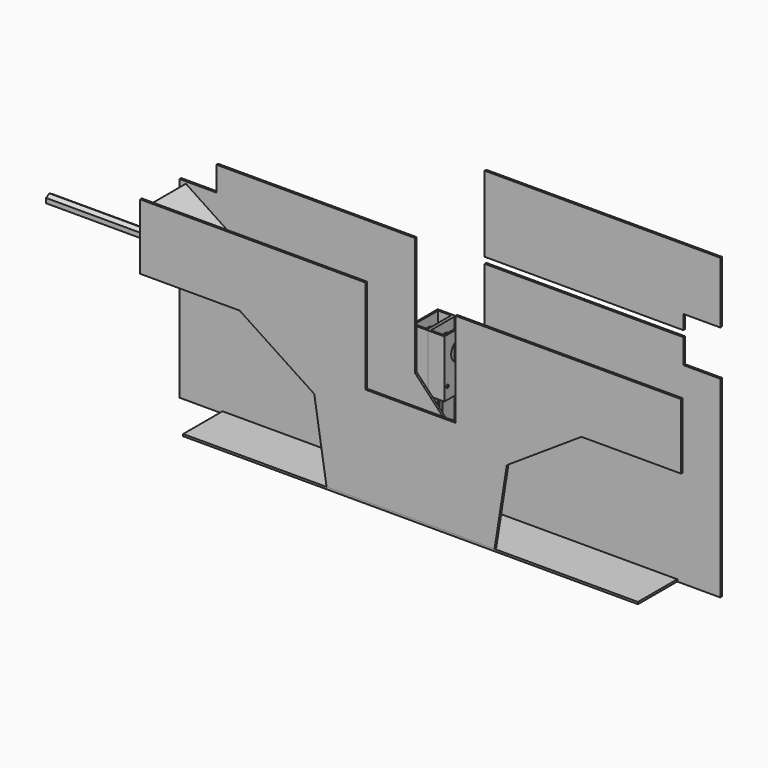
from build123d import *

# Parameters (mm, degrees)
F1_DEPTH  = 3.175
F2_W      = 704.85
F2_H      = 76.2
F3_DEPTH  = 3.175
F0_W      = 365.125
F0_H      = 117.475
F4_DEPTH  = 3.175
F6_DEPTH  = 3.175
F8_DEPTH  = 69.85
F10_DEPTH = 69.85
F11_W     = 25.4
F11_H     = 50.8
F11_W_2   = 20.32
F11_H_2   = 45.72
F12_DEPTH = 88.9
F13_R     = 15.24
F13_R_2   = 2.4003
F14_DEPTH = 25.4
F16_DEPTH = 609.6
F17_W     = 57.15
F17_H     = 38.1
F17_H_2   = 31.75
F18_DEPTH = 3.175
F20_DEPTH = 12.7
F22_DEPTH = 50.8
F23_R     = 15.24
F24_DEPTH = 25.4
F25_W     = 20.32
F25_H     = 45.72
F26_DEPTH = 139.7


# Not quite as in the source:
# - a length typed as a fraction of an inch, garbled in the dataset ("3 / 203.2 mm" for 3/8 in), is restored


with BuildPart() as f1:
    # F0 (on Front) → F1 (new body)
    with BuildSketch(Plane.XZ):
        Polygon((0, 184.15), (-365.125, 184.15), (-365.125, -152.4), (473.075, -152.4), (473.075, 184.15), (107.95, 184.15), (107.95, 0), (53.975, -57.15), (0, 0), align=None)
    extrude(amount=F1_DEPTH)


with BuildPart() as f3:
    # F2 (on face) → F3 (new body)
    with BuildSketch(Plane(origin=(0, 0, -152.4), x_dir=(1, 0, 0), z_dir=(0, 0, -1))):
        with Locations((53.9782664609, 41.275)):
            Rectangle(F2_W, F2_H)
    extrude(amount=-F3_DEPTH)


with BuildPart() as f4:
    # F0 (on Front) → F4 (new body)
    with BuildSketch(Plane.XZ):
        with Locations((290.5125, 252.4125)):
            Rectangle(F0_W, F0_H)
    extrude(amount=F4_DEPTH)


with BuildPart() as f6:
    # F5 (on face) → F6 (new body)
    with BuildSketch(Plane.XZ.offset(79.375)):
        Polygon((-15.875, 3.175), (-15.875, 149.225), (-365.125, 149.225), (-210.9107142857, 47.625), (-95.25, -28.575), (-76.2, -149.225), (184.15, -149.225), (203.2, -28.575), (318.8607142857, 47.625), (473.075, 149.225), (123.825, 149.225), (123.825, 3.175), align=None)
        Polygon((-210.9107142857, 47.625), (-365.125, 149.225), (-365.125, 47.625), align=None)
        Polygon((473.075, 47.625), (473.075, 149.225), (318.8607142857, 47.625), align=None)
    extrude(amount=-F6_DEPTH)


with BuildPart() as f8:
    # F7 (on face) → F8 (new body)
    with BuildSketch(Plane(origin=(0, -76.2, 0), x_dir=(-1, 0, 0), z_dir=(0, 1, 0))):
        Polygon((76.2, -149.225), (95.25, -28.575), (92.1138525851, -28.0798188292), (73.0638525851, -148.7298188292), align=None)
    extrude(amount=F8_DEPTH)


with BuildPart() as f10:
    # F9 (on face) → F10 (new body)
    with BuildSketch(Plane(origin=(0, -76.2, 0), x_dir=(-1, 0, 0), z_dir=(0, 1, 0))):
        Polygon((210.9107142857, 47.625), (354.5197280439, 142.2379972995), (352.7729773688, 144.8893152885), (96.1545673139, -24.1769313358), (97.901317989, -26.8282493249), align=None)
    extrude(amount=F10_DEPTH)


with BuildPart() as f12:
    # F11 (on Top) → F12 (new body)
    with BuildSketch(Plane.XY):
        with Locations((-44.9317730963, 119.1572592371)):
            Rectangle(F11_W, F11_H)
        with Locations((-44.9317730963, 119.1572592371)):
            Rectangle(F11_W_2, F11_H_2, mode=Mode.SUBTRACT)
    extrude(amount=-F12_DEPTH)

    # F13 (on face) → F14 (cut, through all)
    with BuildSketch(Plane(origin=(-57.6317730963, 0, 0), x_dir=(0, -1, 0), z_dir=(-1, 0, 0))):
        with Locations((-122.3322592371, -30.1625)):
            Circle(F13_R)
        with Locations((-100.1072592371, -70.46214)):
            Circle(F13_R_2)
    extrude(amount=-F14_DEPTH, mode=Mode.SUBTRACT)

    # F21 (on face) → F22 (join)
    with BuildSketch(Plane(origin=(0, 0, -88.9), x_dir=(1, 0, 0), z_dir=(0, 0, -1))):
        Polygon((-34.7717730963, -142.0172592371), (-55.0917730963, -142.0172592371), (-55.0917730963, -119.1572592371), (-57.6317730963, -119.1572592371), (-57.6317730963, -144.5572592371), (-32.2317730963, -144.5572592371), (-32.2317730963, -119.1572592371), (-34.7717730963, -119.1572592371), align=None)
    extrude(amount=F22_DEPTH)


with BuildPart() as f16:
    # F15 (on face) → F16 (new body)
    with BuildSketch(Plane(origin=(-57.6317730963, 0, 0), x_dir=(0, -1, 0), z_dir=(-1, 0, 0))):
        Polygon((-122.3322592371, -37.4948484187), (-115.9822592371, -33.8286742094), (-115.9822592371, -26.4963257906), (-122.3322592371, -22.8301515813), (-128.6822592371, -26.4963257906), (-128.6822592371, -33.8286742094), align=None)
    extrude(amount=F16_DEPTH)


with BuildPart() as f18_tool:
    # F17 (on face) → F18 (new body, through all)
    with BuildSketch(Plane.XZ):
        with Locations((444.5, 165.1)):
            Rectangle(F17_W, F17_H)
        with Locations((444.5, 200.025)):
            Rectangle(F17_W, F17_H_2)
        with Locations((-336.55, 165.1)):
            Rectangle(F17_W, F17_H)
    extrude(amount=F18_DEPTH)


with BuildPart() as f1_1:
    add(f1.part)

    # F18: cut by f18_tool
    add(f18_tool.part, mode=Mode.SUBTRACT)


with BuildPart() as f4_1:
    add(f4.part)

    # F18: cut by f18_tool
    add(f18_tool.part, mode=Mode.SUBTRACT)


with BuildPart() as f20:
    # F19 (on Top) → F20 (new body)
    with BuildSketch(Plane.XY):
        Polygon((-451.7894704658, 231.1321839183), (-453.0594704658, 231.1321839183), (-453.0594704658, 204.4621839183), (-376.8594704658, 204.4621839183), (-376.8594704658, 205.7321839183), (-451.7894704658, 205.7321839183), align=None)
    extrude(amount=F20_DEPTH)


with BuildPart() as f24:
    # F23 (on face) → F24 (new body)
    with BuildSketch(Plane(origin=(-57.6317730963, 0, 0), x_dir=(0, -1, 0), z_dir=(-1, 0, 0))):
        Polygon((-119.1572592371, -139.7), (-119.1572592371, -88.9), (-93.7572592371, -88.9), (-93.7572592371, 0), (-144.5572592371, 0), (-144.5572592371, -139.7), align=None)
        with Locations((-122.3322592371, -30.1625)):
            Circle(F23_R, mode=Mode.SUBTRACT)
    extrude(amount=F24_DEPTH)

    # F25 (on face) → F26 (cut, through all)
    with BuildSketch(Plane.XY):
        with Locations((-70.3317730963, 119.1572592371)):
            Rectangle(F25_W, F25_H)
    extrude(amount=-F26_DEPTH, mode=Mode.SUBTRACT)


solid = Compound([f3.part, f6.part, f8.part, f10.part, f12.part, f16.part, f1_1.part, f4_1.part, f20.part, f24.part])
